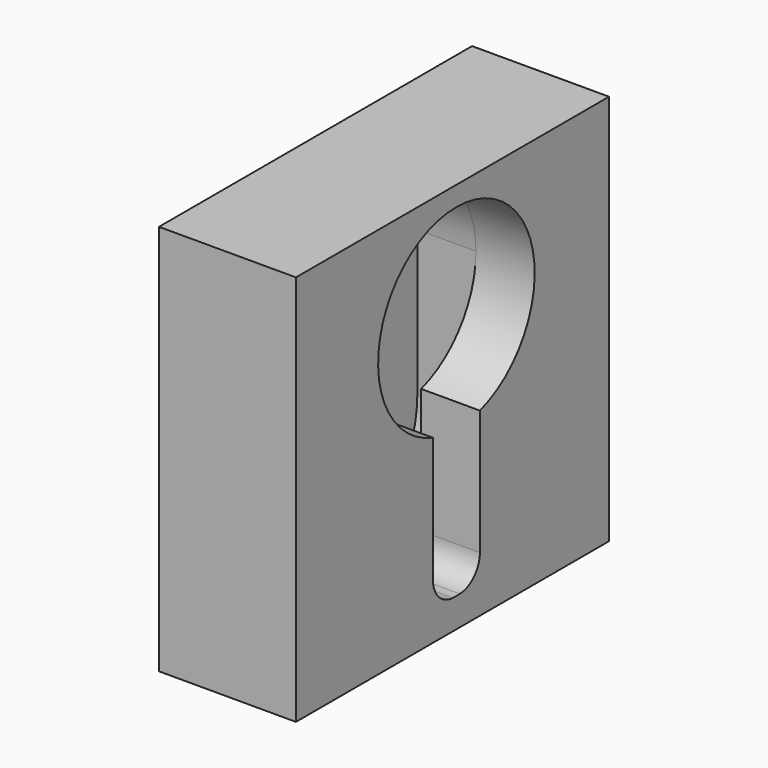
from build123d import *

# Parameters (mm, degrees)
F0_W     = 7
F0_H     = 20
F1_DEPTH = 20
F3_DEPTH = 6
F4_W     = 36.7105286568
F4_H     = 22.0389235765
F5_DEPTH = 3
F6_W     = 20
F6_H     = 20
F7_DEPTH = 3


# Not quite as in the source:
# - after a boolean that leaves OpenCascade's solid faulty, fix() repairs it


with BuildPart() as f1:
    # F0 (on Top) → F1 (new body)
    with BuildSketch(Plane.XY):
        with Locations((-6.9235885665, -0.25)):
            Rectangle(F0_W, F0_H)
    extrude(amount=F1_DEPTH)

    # F2 (on face) → F3 (cut)
    with BuildSketch(Plane.YZ.offset(-3.4235885665)):
        with BuildLine():
            Line((5, 6.5), (5, 14))
            ThreePointArc((5, 14), (0, 19), (-5, 14))
            Line((-5, 14), (-5, 6.5))
            ThreePointArc((-5, 6.5), (-3.5355339059, 2.9644660941), (0, 1.5))
            ThreePointArc((0, 1.5), (3.5355339059, 2.9644660941), (5, 6.5))
        make_face()
    extrude(amount=-F3_DEPTH, mode=Mode.SUBTRACT)

    # F4 (on face) → F5 (cut)
    with BuildSketch(Plane.YZ.offset(-3.4235885665)):
        with Locations((-1.3269511983, 11.0194617882)):
            Rectangle(F4_W, F4_H)
    extrude(amount=-F5_DEPTH, mode=Mode.SUBTRACT)

    # F6 (on face) → F7 (join)
    with BuildSketch(Plane.YZ.offset(-6.4235885665)):
        with Locations((-0.25, 10)):
            Rectangle(F6_W, F6_H)
        with BuildLine():
            ThreePointArc((-1.5, 9.2303039929), (0, 19), (1.5, 9.2303039929))
            Line((1.5, 9.2303039929), (1.5, 2.8392676962))
            ThreePointArc((1.5, 2.8392676962), (1.1297736268, 1.9163028593), (0.2243504639, 1.505035849))
            ThreePointArc((0.2243504639, 1.505035849), (0, 1.5), (-0.2243504639, 1.505035849))
            ThreePointArc((-0.2243504639, 1.505035849), (-1.1297736268, 1.9163028593), (-1.5, 2.8392676962))
            Line((-1.5, 2.8392676962), (-1.5, 9.2303039929))
        make_face(mode=Mode.SUBTRACT)
    extrude(amount=F7_DEPTH)

    add(f1.part.fix(), mode=Mode.REPLACE)


solid = f1.part
